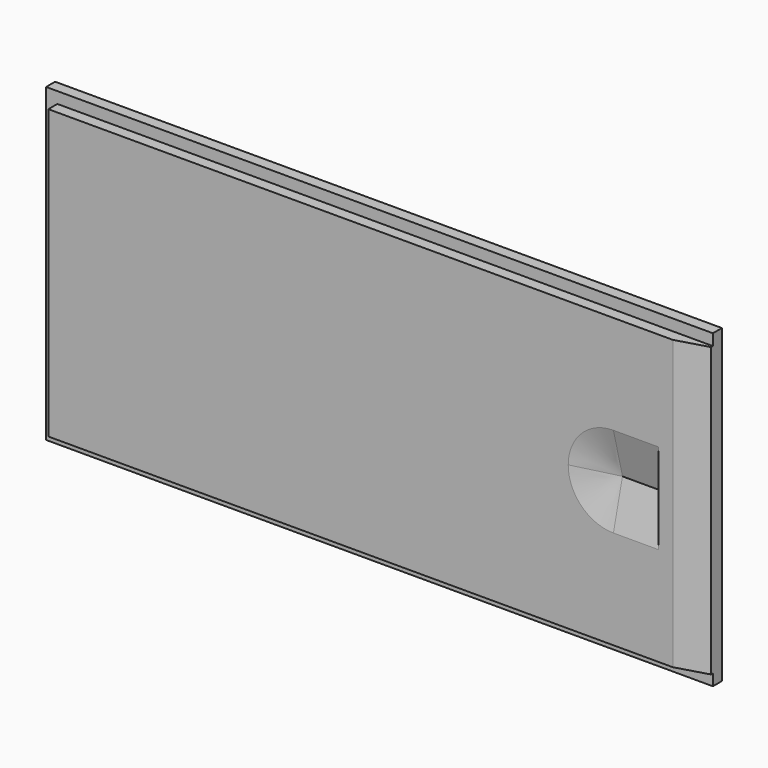
from build123d import *

# Parameters (mm, degrees)
F0_W     = 374.65
F0_H     = 174.625
F1_DEPTH = 12.7
F2_W     = 350.8375
F2_H     = 6.35
F2_W_2   = 6.35
F2_H_2   = 161.925
F2_W_3   = 17.4625
F3_DEPTH = 6.35
F4_SIZE2 = 5.08
F4_SIZE  = 17.4625
F2_W_4   = 50.8
F2_H_3   = 50.8
F5_DEPTH = 6.35
F6_R     = 25.39999
F7_SIZE2 = 6.34999
F7_SIZE  = 25.39999


# Not quite as in the source:
# - a fillet or chamfer is up to 0.001 mm smaller than in the source, because OpenCascade refuses the exact size


with BuildPart() as f1:
    # F0 (on Front) → F1 (new body)
    with BuildSketch(Plane.XZ):
        Rectangle(F0_W, F0_H)
    extrude(amount=F1_DEPTH)

    # F2 (on face) → F3 (cut)
    with BuildSketch(Plane.XZ.offset(12.7)):
        with Locations((-5.55625, 84.1375)):
            Rectangle(F2_W, F2_H)
        with Locations((-184.15, 84.1375)):
            Rectangle(F2_W_2, F2_H)
        with Locations((-184.15, 0)):
            Rectangle(F2_W_2, F2_H_2)
        with Locations((-184.15, -84.1375)):
            Rectangle(F2_W_2, F2_H)
        with Locations((-5.55625, -84.1375)):
            Rectangle(F2_W, F2_H)
        with Locations((178.59375, -84.1375)):
            Rectangle(F2_W_3, F2_H)
        with Locations((178.59375, 84.1375)):
            Rectangle(F2_W_3, F2_H)
    extrude(amount=-F3_DEPTH, mode=Mode.SUBTRACT)

    # F4
    f4_edges = [f1.edges().sort_by_distance(p)[0] for p in [
        (187.325, -12.7, 0),
    ]]
    f4_side = f1.faces().sort_by_distance((3.175, -12.7, 0))[0]
    chamfer(f4_edges, length=F4_SIZE, length2=F4_SIZE2, reference=f4_side)

    # F2 (on face) → F5 (cut)
    with BuildSketch(Plane.XZ.offset(12.7)):
        with Locations((136.525, 0)):
            Rectangle(F2_W_4, F2_H_3)
    extrude(amount=-F5_DEPTH, mode=Mode.SUBTRACT)

    # F6 (radius 25.4 in the source; OpenCascade refuses exactly that, so slightly less here)
    f6_edges = [f1.edges().sort_by_distance(p)[0] for p in [
        (111.125, -9.525, -25.4),
        (111.125, -9.525, 25.4),
    ]]
    fillet(f6_edges, radius=F6_R)

    # F7 (size 25.4 and 6.35 in the source; OpenCascade refuses exactly that, so slightly less here)
    f7_edges = [f1.edges().sort_by_distance(p)[0] for p in [
        (118.564485, -6.35, -17.960515),
    ]]
    f7_side = f1.faces().sort_by_distance((138.896085, -6.35, 0))[0]
    chamfer(f7_edges, length=F7_SIZE, length2=F7_SIZE2, reference=f7_side)


solid = f1.part
